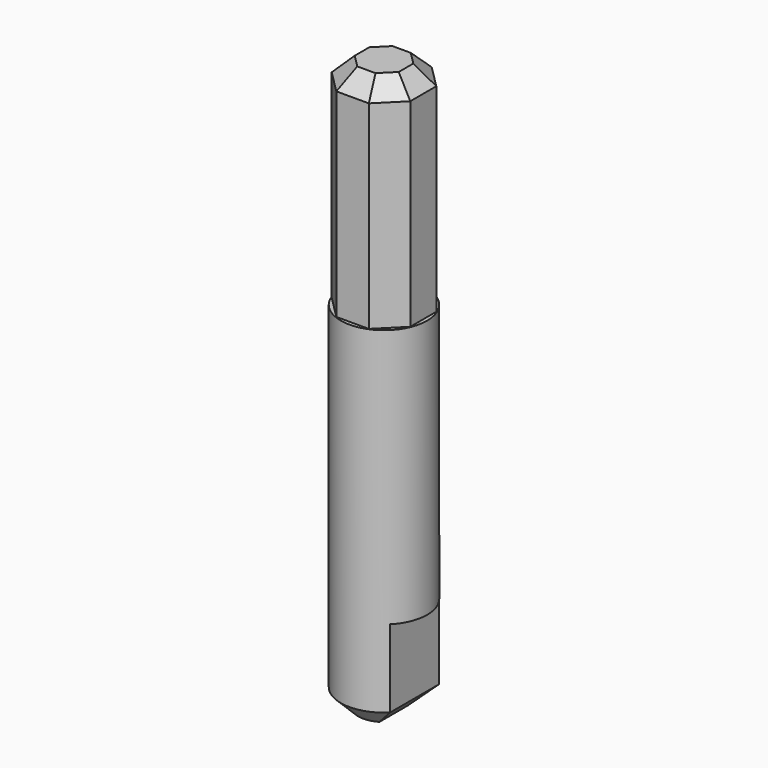
from build123d import *

# Parameters (mm, degrees)
F0_R         = 5
F1_DEPTH     = 66
F2_R         = 5
F3_DEPTH     = 25
F5_DEPTH     = 11
F6_T1_DEPTH  = 14.0560753695
F6_T3_DEPTH  = 14.0560753695
F6_T5_DEPTH  = 14.0560753695
F6_T7_DEPTH  = 14.0560753695
F6_T9_DEPTH  = 14.0560753695
F6_T11_DEPTH = 14.0560753695
F6_T13_DEPTH = 17.3577997637
F6_T15_DEPTH = 17.3577997637
F6_T18_ANGLE = 298.0668340959


# Not quite as in the source:
# - a fillet or chamfer that OpenCascade refuses, or shapes differently, is made with other operations: its cross-section is extruded or revolved along the edge and cut away or added


with BuildPart() as f1:
    # F0 (on Top) → F1 (new body)
    with BuildSketch(Plane.XY):
        Circle(F0_R)
    extrude(amount=F1_DEPTH)

    # F2 (on face) → F3 (cut)
    with BuildSketch(Plane.XY.offset(66)):
        Circle(F2_R)
        Polygon((4.55, 1.8846717088), (4.55, -1.8846717088), (1.8846717088, -4.55), (-1.8846717088, -4.55), (-4.55, -1.8846717088), (-4.55, 1.8846717088), (-1.8846717088, 4.55), (1.8846717088, 4.55), align=None, mode=Mode.SUBTRACT)
    extrude(amount=-F3_DEPTH, mode=Mode.SUBTRACT)

    # F4 (on face) → F5 (cut)
    with BuildSketch(Plane(origin=(0, 0, 0), x_dir=(1, 0, 0), z_dir=(0, 0, -1))):
        with BuildLine():
            ThreePointArc((5, 0), (4.6193976626, 1.9134171618), (3.5355339059, 3.5355339059))
            Line((3.5355339059, 3.5355339059), (3.5355339059, -3.5355339059))
            ThreePointArc((3.5355339059, -3.5355339059), (4.6193976626, -1.9134171618), (5, 0))
        make_face()
        with BuildLine():
            ThreePointArc((-3.5355339059, -3.5355339059), (0, -5), (3.5355339059, -3.5355339059))
            Line((3.5355339059, -3.5355339059), (-3.5355339059, -3.5355339059))
        make_face()
    extrude(amount=-F5_DEPTH, mode=Mode.SUBTRACT)

    # F6: chamfer of 2 on 11 edges, made by hand

    # F6_s2 → F6_t1 (cut)
    with BuildSketch(Plane(origin=(-4.9695731053, 4.9695731053, 0), x_dir=(0, 0, 1), z_dir=(0.7071067812, -0.7071067812, 0))):
        Polygon((64, -4.55), (66, -2.55), (66, -4.55), align=None)
    extrude(amount=F6_T1_DEPTH, mode=Mode.SUBTRACT)

    # F6_s4 → F6_t3 (cut)
    with BuildSketch(Plane.XZ.offset(-7.0280376847)):
        Polygon((4.55, 64), (2.55, 66), (4.55, 66), align=None)
        Polygon((-4.55, 64), (-2.55, 66), (-4.55, 66), align=None)
    extrude(amount=F6_T3_DEPTH, mode=Mode.SUBTRACT)

    # F6_s6 → F6_t5 (cut)
    with BuildSketch(Plane(origin=(4.9695731053, 4.9695731053, 0), x_dir=(0, 0, 1), z_dir=(-0.7071067812, -0.7071067812, 0))):
        Polygon((64, -4.55), (66, -2.55), (66, -4.55), align=None)
    extrude(amount=F6_T5_DEPTH, mode=Mode.SUBTRACT)

    # F6_s8 → F6_t7 (cut)
    with BuildSketch(Plane.YZ.offset(-7.0280376847)):
        Polygon((-4.55, 64), (-2.55, 66), (-4.55, 66), align=None)
        Polygon((4.55, 64), (2.55, 66), (4.55, 66), align=None)
    extrude(amount=F6_T7_DEPTH, mode=Mode.SUBTRACT)

    # F6_s10 → F6_t9 (cut)
    with BuildSketch(Plane(origin=(4.9695731053, -4.9695731053, 0), x_dir=(0, 0, 1), z_dir=(-0.7071067812, 0.7071067812, 0))):
        Polygon((64, -4.55), (66, -2.55), (66, -4.55), align=None)
    extrude(amount=F6_T9_DEPTH, mode=Mode.SUBTRACT)

    # F6_s12 → F6_t11 (cut)
    with BuildSketch(Plane(origin=(-4.9695731053, -4.9695731053, 0), x_dir=(0, 0, 1), z_dir=(0.7071067812, 0.7071067812, 0))):
        Polygon((64, -4.55), (66, -2.55), (66, -4.55), align=None)
    extrude(amount=F6_T11_DEPTH, mode=Mode.SUBTRACT)

    # F6_s14 → F6_t13 (cut)
    with BuildSketch(Plane.XZ.offset(-8.6788998819)):
        Polygon((3.5355339059, 2), (1.5355339059, 0), (3.5355339059, 0), align=None)
    extrude(amount=F6_T13_DEPTH, mode=Mode.SUBTRACT)

    # F6_s16 → F6_t15 (cut)
    with BuildSketch(Plane.YZ.offset(-8.6788998819)):
        Polygon((3.5355339059, 2), (1.5355339059, 0), (3.5355339059, 0), align=None)
    extrude(amount=F6_T15_DEPTH, mode=Mode.SUBTRACT)

    # F6_s17 → F6_t18 (revolve, cut)
    with BuildSketch(Plane(origin=(0, 0, 0), x_dir=(0, 0, 1), z_dir=(0.9701544633, -0.2424877673, 0))):
        Polygon((2, -5), (0, -3), (0, -5), align=None)
    revolve(axis=Axis((0, 0, 0), (0, 0, 1)), revolution_arc=F6_T18_ANGLE, mode=Mode.SUBTRACT)


solid = f1.part
